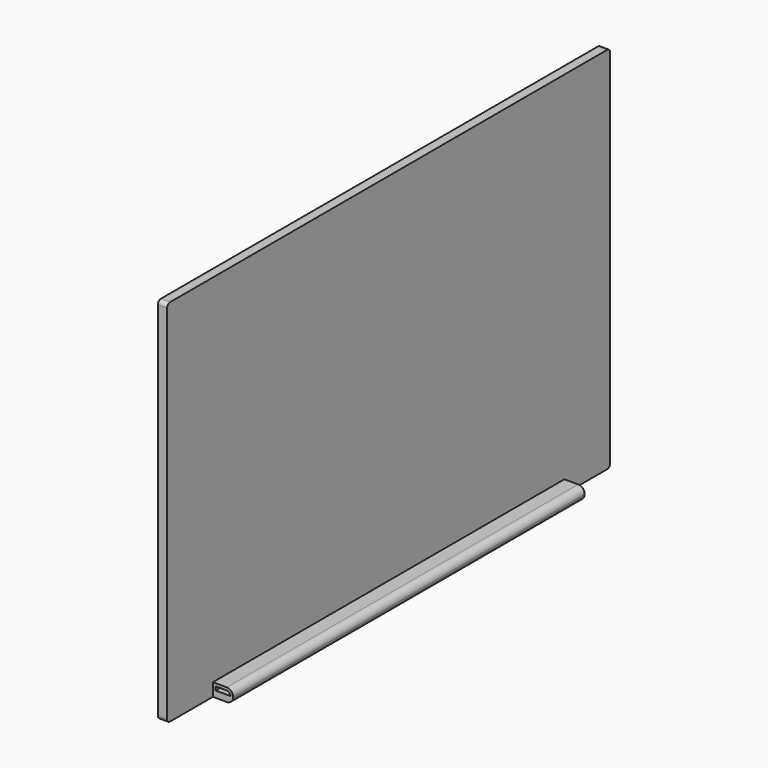
from build123d import *

# Parameters (mm, degrees)
F0_W     = 5
F0_H     = 200
F1_DEPTH = 300
F2_W     = 11
F2_H     = 7
F3_DEPTH = 300
F4_R     = 3.49999
F5_W     = 15
F5_H     = 31
F6_DEPTH = 7.001
F7_R     = 2
F8_W     = 8
F8_H     = 2
F9_DEPTH = 27
F10_R    = 1.99999


# Not quite as in the source:
# - a fillet or chamfer is up to 0.001 mm smaller than in the source, because OpenCascade refuses the exact size


with BuildPart() as f1:
    # F0 (on Front) → F1 (new body)
    with BuildSketch(Plane.XZ):
        with Locations((2.5, 100)):
            Rectangle(F0_W, F0_H)
    extrude(amount=F1_DEPTH)

    # F2 (on face) → F3 (join)
    with BuildSketch(Plane.XZ.offset(300)):
        with Locations((10.5, 3.5)):
            Rectangle(F2_W, F2_H)
    extrude(amount=-F3_DEPTH)

    # F4 (radius 3.5 in the source; OpenCascade refuses exactly that, so slightly less here)
    f4_edges = [f1.edges().sort_by_distance(p)[0] for p in [
        (16, -150, 7),
        (16, -150, 0),
    ]]
    fillet(f4_edges, radius=F4_R)

    # F5 (on face) → F6 (cut, through all)
    with BuildSketch(Plane.XY.offset(7)):
        with Locations((12.5, -284.5)):
            Rectangle(F5_W, F5_H)
        with Locations((12.5, -15.5)):
            Rectangle(F5_W, F5_H)
    extrude(amount=-F6_DEPTH, mode=Mode.SUBTRACT)

    # F7
    f7_edges = [f1.edges().sort_by_distance(p)[0] for p in [
        (2.5, -300, 200),
        (2.5, 0, 200),
        (2.5, -300, 0),
        (2.5, 0, 0),
    ]]
    fillet(f7_edges, radius=F7_R)

    # F8 (on face) → F9 (cut)
    with BuildSketch(Plane.XZ.offset(269)):
        with Locations((10.5, 4.5)):
            Rectangle(F8_W, F8_H)
    extrude(amount=-F9_DEPTH, mode=Mode.SUBTRACT)

    # F10 (radius 2 in the source; OpenCascade refuses exactly that, so slightly less here)
    f10_edges = [f1.edges().sort_by_distance(p)[0] for p in [
        (14.5, -255.5, 5.5),
    ]]
    fillet(f10_edges, radius=F10_R)


solid = f1.part
